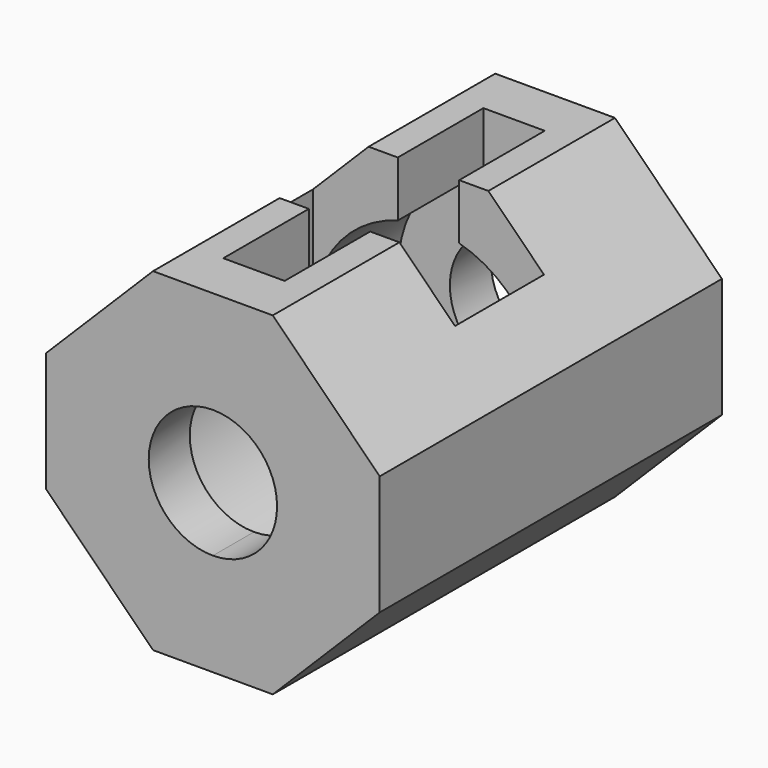
from build123d import *

# Parameters (mm, degrees)
F3_W          = 7.8
F3_H          = 10
F3_W_2        = 5.4
F3_H_2        = 2.6
F4_DEPTH      = 7.8
F7_DEPTH      = 3.8
F7_DEPTH_BACK = 3.8
F8_W          = 5.4
F8_H          = 2.6
F9_DEPTH      = 3.9
F10_W         = 1.4347932888
F10_H         = 7.6
F11_DEPTH     = 3.9
F13_DEPTH     = 10.001
F14_T1_DEPTH  = 22.8584149398


# Not quite as in the source:
# - a fillet or chamfer that OpenCascade refuses, or shapes differently, is made with other operations: its cross-section is extruded or revolved along the edge and cut away or added


with BuildPart() as f4:
    # F3 (on Top) → F4 (new body)
    with BuildSketch(Plane.XY):
        Rectangle(F3_W, F3_H)
        Rectangle(F3_W_2, F3_H_2, mode=Mode.SUBTRACT)
        Rectangle(F3_W_2, F3_H_2)
    extrude(amount=F4_DEPTH)

    # F6 (on offset) → F7 (cut, two sides)
    with BuildSketch(Plane.XZ) as f7_sk:
        with BuildLine():
            ThreePointArc((0, 1.2), (1.9091883092, 1.9908116908), (2.7, 3.9))
            ThreePointArc((2.7, 3.9), (1.9091883092, 5.8091883092), (0, 6.6))
            Line((0, 6.6), (0, 3.9))
            Line((0, 3.9), (0, 1.2))
        make_face()
        with BuildLine():
            Line((0, 3.9), (0, 6.6))
            ThreePointArc((0, 6.6), (-2.7, 3.9), (0, 1.2))
            Line((0, 1.2), (0, 3.9))
        make_face()
    extrude(amount=-F7_DEPTH, mode=Mode.SUBTRACT)
    extrude(f7_sk.sketch, amount=F7_DEPTH_BACK, mode=Mode.SUBTRACT)

    # F8 (on face) → F9 (cut)
    with BuildSketch(Plane.XY.offset(7.8)):
        Rectangle(F8_W, F8_H)
    extrude(amount=-F9_DEPTH, mode=Mode.SUBTRACT)

    # F10 (on face) → F11 (cut)
    with BuildSketch(Plane.XY.offset(7.8)):
        Rectangle(F10_W, F10_H)
    extrude(amount=-F11_DEPTH, mode=Mode.SUBTRACT)

    # F12 (on face) → F13 (cut, through all)
    with BuildSketch(Plane.XZ.offset(5)):
        with BuildLine():
            ThreePointArc((0, 2.4), (1.0606601718, 2.8393398282), (1.5, 3.9))
            ThreePointArc((1.5, 3.9), (1.0606601718, 4.9606601718), (0, 5.4))
            Line((0, 5.4), (0, 3.9))
            Line((0, 3.9), (0, 2.4))
        make_face()
        with BuildLine():
            Line((0, 3.9), (0, 5.4))
            ThreePointArc((0, 5.4), (-1.5, 3.9), (0, 2.4))
            Line((0, 2.4), (0, 3.9))
        make_face()
    extrude(amount=-F13_DEPTH, mode=Mode.SUBTRACT)

    # F14: chamfer of 2.5 on 4 edges, made by hand

    # F14_s2 → F14_t1 (cut)
    with BuildSketch(Plane.XZ.offset(-11.4292074699)):
        Polygon((-1.4, 7.8), (-3.9, 5.3), (-3.9, 7.8), align=None)
        Polygon((-1.4, 0), (-3.9, 2.5), (-3.9, 0), align=None)
        Polygon((3.9, 2.5), (1.4, 0), (3.9, 0), align=None)
        Polygon((3.9, 5.3), (1.4, 7.8), (3.9, 7.8), align=None)
    extrude(amount=F14_T1_DEPTH, mode=Mode.SUBTRACT)


solid = f4.part
